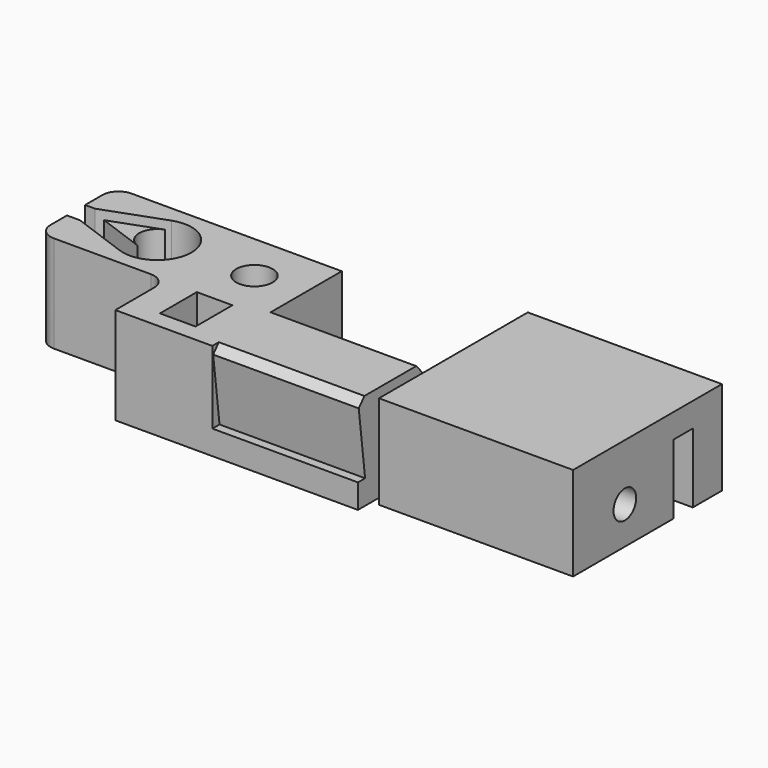
from build123d import *

# Parameters (mm, degrees)
F1_DEPTH  = 12
F3_DEPTH  = 18
F4_SIZE   = 1
F5_D      = 4.5
F6_R      = 1.75
F7_DEPTH  = 35
F8_W      = 4.4
F8_H      = 5.7
F9_DEPTH  = 8
F11_DEPTH = 8
F14_DEPTH = 24
F15_W     = 14
F15_H     = 11.6
F16_DEPTH = 6
F17_R     = 1.75
F18_DEPTH = 6
F20_DEPTH = 8.6


with BuildPart() as f1:
    # F0 (on Top) → F1 (new body)
    with BuildSketch(Plane.XY):
        with BuildLine():
            ThreePointArc((-10, -4), (-9.4142135624, -5.4142135624), (-8, -6))
            Line((-8, -6), (4, -6))
            ThreePointArc((4, -6), (5.4142135624, -6.5857864376), (6, -8))
            Line((6, -8), (6, -14))
            Line((6, -14), (36, -14))
            Line((36, -14), (36, -6))
            Line((36, -6), (36, -4))
            Line((36, -4), (18, -4))
            Line((18, -4), (18, 6))
            Line((18, 6), (-8, 6))
            ThreePointArc((-8, 6), (-9.4142135624, 5.4142135624), (-10, 4))
            Line((-10, 4), (-10, -4))
        make_face()
    extrude(amount=F1_DEPTH)

    # F2 (on face) → F3 (cut, through all)
    with BuildSketch(Plane.YZ.offset(36)):
        Polygon((-12.8949389519, 3), (-14, 12), (-16, 12), (-16, 3), align=None)
        Polygon((-2, 3), (-2, 12), (-4, 12), (-5.1050610481, 3), align=None)
    extrude(amount=-F3_DEPTH, mode=Mode.SUBTRACT)

    # F4
    f4_edges = [f1.edges().sort_by_distance(p)[0] for p in [
        (27, -14, 12),
        (27, -4, 12),
    ]]
    chamfer(f4_edges, length=F4_SIZE)

    # F5 (through all)
    with Locations(Plane(origin=(0, 0, 0), x_dir=(1, 0, 0), z_dir=(0, 0, -1))):
        with Locations((0, 0), (12, 0)):
            Hole(F5_D / 2)

    # F6 (on face) → F7 (cut)
    with BuildSketch(Plane.YZ.offset(36)):
        with Locations((-9, 8)):
            Circle(F6_R)
    extrude(amount=-F7_DEPTH, mode=Mode.SUBTRACT)

    # F8 (on face) → F9 (cut)
    with BuildSketch(Plane.XY.offset(12)):
        with Locations((12, -9)):
            Rectangle(F8_W, F8_H)
    extrude(amount=-F9_DEPTH, mode=Mode.SUBTRACT)

    # F10 (on face) → F11 (cut)
    with BuildSketch(Plane.XY.offset(12)):
        with BuildLine():
            Line((-10.71459784, -1.4658419218), (-8.39880112, -1.4658419218))
            Line((-8.39880112, -1.4658419218), (-1.4683823551, -3.9883080632))
            ThreePointArc((-1.4683823551, -3.9883080632), (4.2275118557, 0), (-1.4683823551, 3.9883080632))
            Line((-1.4683823551, 3.9883080632), (-8.759381076, 1.3346015508))
            Line((-8.759381076, 1.3346015508), (-10.71459784, 1.3346015508))
            Line((-10.71459784, 1.3346015508), (-10.71459784, -1.4658419218))
        make_face()
        with BuildLine():
            Line((-6.5785599004, 0), (-0.7695453225, 2.1143083968))
            ThreePointArc((-0.7695453225, 2.1143083968), (2.25, 0), (-0.7695453225, -2.1143083968))
            Line((-0.7695453225, -2.1143083968), (-6.5785599004, 0))
        make_face(mode=Mode.SUBTRACT)
    extrude(amount=-F11_DEPTH, mode=Mode.SUBTRACT)


with BuildPart() as f14:
    # F13 (on offset) → F14 (new body)
    with BuildSketch(Plane.YZ.offset(41)):
        with BuildLine():
            Line((-13.1455547413, 3.4), (-14.0550757095, 10.8074538484))
            ThreePointArc((-14.0550757095, 10.8074538484), (-13.79613929, 11.6413654001), (-13, 12))
            Line((-13, 12), (-5, 12))
            ThreePointArc((-5, 12), (-4.20386071, 11.6413654001), (-3.9449242905, 10.8074538484))
            Line((-3.9449242905, 10.8074538484), (-4.8544452587, 3.4))
            Line((-4.8544452587, 3.4), (-4, 3.4))
            Line((-4, 3.4), (6, 3.4))
            Line((6, 3.4), (6, 15))
            Line((6, 15), (-17, 15))
            Line((-17, 15), (-17, 3.4))
            Line((-17, 3.4), (-14, 3.4))
            Line((-14, 3.4), (-13.1455547413, 3.4))
        make_face()
    extrude(amount=F14_DEPTH)

    # F15 (on face) → F16 (join)
    with BuildSketch(Plane.YZ.offset(65)):
        with Locations((-10, 9.2)):
            Rectangle(F15_W, F15_H)
    extrude(amount=-F16_DEPTH)

    # F17 (on face) → F18 (cut, through all)
    with BuildSketch(Plane.YZ.offset(65)):
        with Locations((-9, 8)):
            Circle(F17_R)
    extrude(amount=-F18_DEPTH, mode=Mode.SUBTRACT)

    # F19 (on face) → F20 (cut, through all)
    with BuildSketch(Plane(origin=(0, 0, 3.4), x_dir=(1, 0, 0), z_dir=(0, 0, -1))):
        with BuildLine():
            Line((60.9248853567, 1.5), (53.9058666579, 3.380740392))
            ThreePointArc((53.9058666579, 3.380740392), (49.5, 0), (53.9058666579, -3.380740392))
            Line((53.9058666579, -3.380740392), (60.9248853567, -1.5))
            Line((60.9248853567, -1.5), (66, -1.5))
            Line((66, -1.5), (66, 1.5))
            Line((66, 1.5), (60.9248853567, 1.5))
        make_face()
        with BuildLine():
            ThreePointArc((53.3882285677, -1.4488887394), (51.5, 0), (53.3882285677, 1.4488887394))
            Line((53.3882285677, 1.4488887394), (58.7955549577, 0))
            Line((58.7955549577, 0), (53.3882285677, -1.4488887394))
        make_face(mode=Mode.SUBTRACT)
    extrude(amount=-F20_DEPTH, mode=Mode.SUBTRACT)


solid = Compound([f1.part, f14.part])
